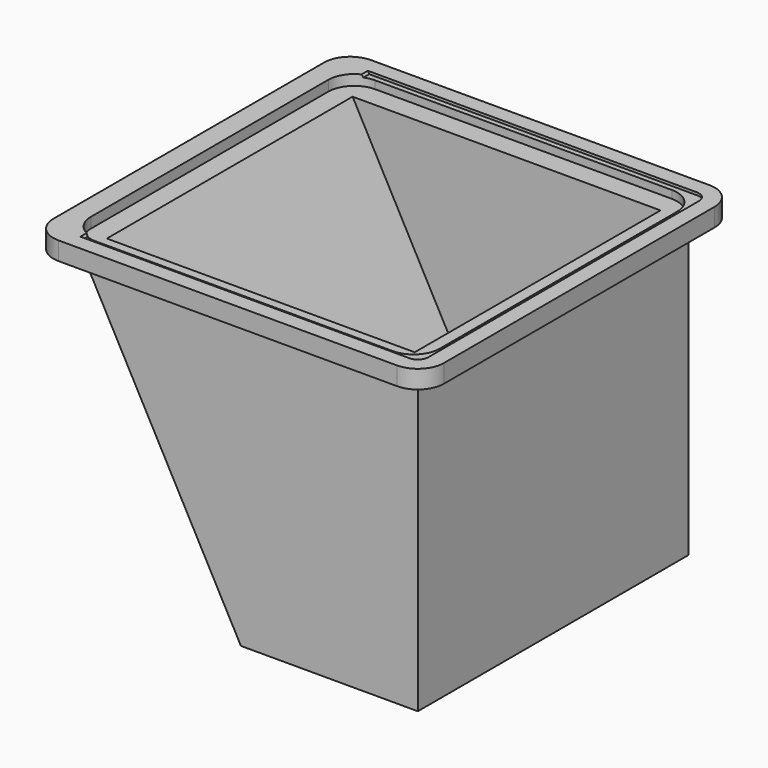
from build123d import *

# Parameters (mm, degrees)
F0_W        = 75
F0_H        = 75
F1_DEPTH    = 3.5
F2_W        = 65
F2_H        = 65
F3_DEPTH    = 3.5
F4_R        = 5
F6_DEPTH    = 65
F7_T        = 3
F7_T3_DEPTH = 70.7303019134
F7_T5_DEPTH = 71
F7_T7_DEPTH = 6.5680995141
F7_T9_DEPTH = 6.5
F8_W        = 67
F8_H        = 67
F9_DEPTH    = 2
F10_R       = 5


# Not quite as in the source:
# - a shell that OpenCascade refuses in one call is made with other operations: the cavity is built on its own and cut out


with BuildPart() as f1:
    # F0 (on Top) → F1 (new body)
    with BuildSketch(Plane.XY):
        with Locations((1.4847200364, -1.2060580678)):
            Rectangle(F0_W, F0_H)
    extrude(amount=F1_DEPTH)

    # F2 (on face) → F3 (cut)
    with BuildSketch(Plane.XY.offset(3.5)):
        with Locations((1.4847200364, -1.2060580678)):
            Rectangle(F2_W, F2_H)
    extrude(amount=-F3_DEPTH, mode=Mode.SUBTRACT)

    # F4
    f4_edges = [f1.edges().sort_by_distance(p)[0] for p in [
        (38.98472, -38.706058, 1.75),
        (-36.01528, -38.706058, 1.75),
        (38.98472, 36.293942, 1.75),
        (-36.01528, 36.293942, 1.75),
    ]]
    fillet(f4_edges, radius=F4_R)

    # F5 (on face) → F6 (join)
    with BuildSketch(Plane(origin=(0, -33.7060580678, 0), x_dir=(-1, 0, 0), z_dir=(0, 1, 0))):
        Polygon((31.0152799636, 3.5), (-33.9847200364, 3.5), (-33.9847200364, -57), (0, -57), (31.0152799636, 0.5), align=None)
    extrude(amount=F6_DEPTH)

    # F7: shell of thickness 3, made by hand


with BuildPart() as f7_core1:
    # F7_t2: copy of F1
    add(f1.part)

    # the walls: a layer under each face that stays
    f7_faces = [f7_core1.faces().sort_by_distance(p)[0] for p in [
        (1.4847200364, 36.2939419322, 1.75),
        (-33.5152799636, -36.2060580678, 0),
        (37.5202539423, 34.8294758382, 1.75),
        (-34.5508138695, 34.8294758382, 1.75),
        (38.9847200364, -1.2060580678, 1.75),
        (-36.0152799636, -1.2060580678, 1.75),
        (37.5202539423, -37.2415919737, 1.75),
        (-34.5508138695, -37.2415919737, 1.75),
        (1.4847200364, -38.7060580678, 1.75),
        (-30.9703302825, -33.7060580678, 0.0833333333),
        (1.6195690797, -33.7060580678, -28.5),
        (33.9847200364, -1.2060580678, -28.5),
        (1.6195690797, 31.2939419322, -28.5),
        (-30.8804309203, 31.2939419322, 0.0833333333),
        (-31.0152799636, -1.2060580678, 0.25),
        (-15.5076399818, -1.2060580678, -28.25),
        (16.9923600182, -1.2060580678, -57),
    ]]
    thicken(f7_faces, amount=-F7_T, mode=Mode.SUBTRACT)

    # F7_s4 → F7_t3 (cut)
    with BuildSketch(Plane.YZ.offset(-33.745581877)):
        Polygon((-33.7360580678, -0.03), (-33.7060580678, 3), (-30.7060580678, 3), (-30.7060580678, 0), align=None)
        Polygon((31.3239419322, -0.03), (31.2939419322, 3), (28.2939419322, 3), (28.2939419322, 0), align=None)
    extrude(amount=F7_T3_DEPTH, mode=Mode.SUBTRACT)

    # F7_s6 → F7_t5 (cut)
    with BuildSketch(Plane.XZ.offset(-34.2939419322)):
        Polygon((34.0147200364, -0.03), (33.9847200364, 3), (30.9847200364, 3), (30.9847200364, 0), align=None)
        Polygon((-31.0116837883, 0.485757878), (-34.0152799636, 0.5), (-34.0152799636, 12.3810577497), (-28.3748974906, 1.9242122019), align=None)
    extrude(amount=F7_T5_DEPTH, mode=Mode.SUBTRACT)

    # F7_s8 → F7_t7 (cut)
    with BuildSketch(Plane(origin=(-5.5050917478, 0, 10.2060267027), x_dir=(0, 1, 0), z_dir=(-0.4747374006, 0, 0.880127491))):
        Polygon((-33.6760580678, 27.0900318369), (-36.7060580678, 27.0600318369), (-36.7060580678, 24.0600318369), (-33.7060580678, 24.0600318369), align=None)
        Polygon((31.2639419322, 27.0900318369), (34.2939419322, 27.0600318369), (34.2939419322, 24.0600318369), (31.2939419322, 24.0600318369), align=None)
    extrude(amount=F7_T7_DEPTH, mode=Mode.SUBTRACT)

    # F7_s10 → F7_t9 (cut)
    with BuildSketch(Plane.XY.offset(-3)):
        Polygon((-30.9852799636, -33.6760580678), (-31.0152799636, -36.7060580678), (-34.0152799636, -36.7060580678), (-34.0152799636, -33.7060580678), align=None)
        Polygon((-30.9852799636, 31.2639419322), (-31.0152799636, 34.2939419322), (-34.0152799636, 34.2939419322), (-34.0152799636, 31.2939419322), align=None)
    extrude(amount=F7_T9_DEPTH, mode=Mode.SUBTRACT)


with BuildPart() as f1_1:
    add(f1.part)

    # what is left inside the walls is the cavity
    f7_cavity = [f7_core1.part.solids().sort_by_distance(p)[0] for p in [
        (3.379924, -12.706058, 3.47),
    ]]
    add(f7_cavity, mode=Mode.SUBTRACT)

    # F8 (on face) → F9 (cut)
    with BuildSketch(Plane.XY.offset(3.5)):
        with Locations((1.4847200364, -1.2060580678)):
            Rectangle(F8_W, F8_H)
    extrude(amount=-F9_DEPTH, mode=Mode.SUBTRACT)

    # F10
    f10_edges = [f1_1.edges().sort_by_distance(p)[0] for p in [
        (-32.01528, 32.293942, 2.5),
        (34.98472, 32.293942, 2.25),
        (-32.01528, -34.706058, 2.5),
        (34.98472, -34.706058, 2.25),
    ]]
    fillet(f10_edges, radius=F10_R)


solid = f1_1.part
